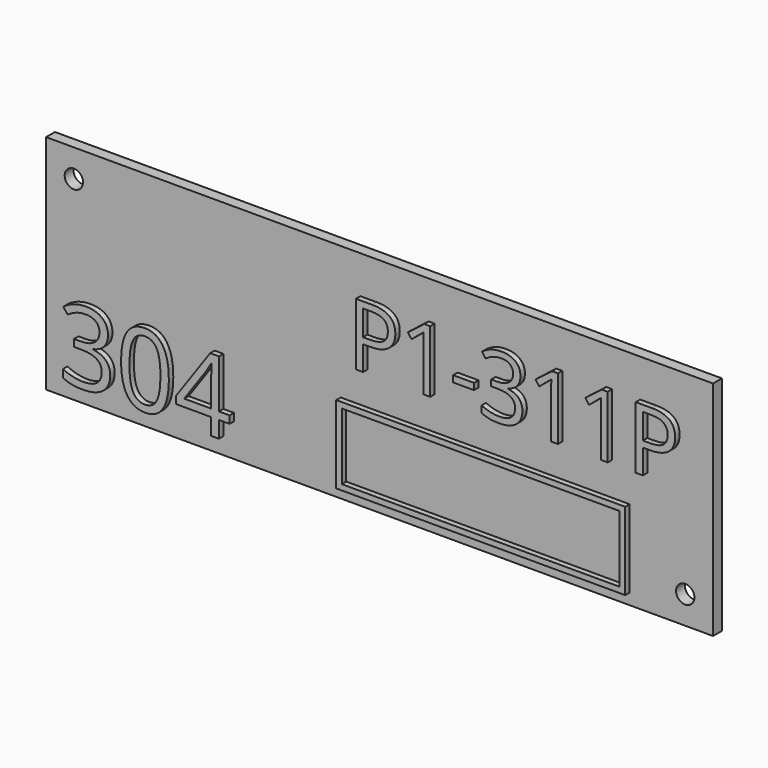
from build123d import *

# Parameters (mm, degrees)
F0_W         = 120
F0_H         = 40
F1_DEPTH     = 2
F3_D         = 3.3
F4_TEXT_SIZE = 15.681149951
F5_DEPTH     = 1
F6_TEXT_SIZE = 18.1818181818
F7_DEPTH     = 1
F8_W         = 52
F8_H         = 14
F8_W_2       = 49.99999962
F8_H_2       = 11.99999962
F9_DEPTH     = 1


# Not quite as in the source:
# - Text() gives the source's letters only with a copy of the font that has no kerning and outlines rounded to 1/6400 em; it was checked with that copy


with BuildPart() as f1:
    # F0 (on Front) → F1 (new body)
    with BuildSketch(Plane.XZ):
        Rectangle(F0_W, F0_H)
    extrude(amount=F1_DEPTH)

    # F3 (through all)
    with Locations(Plane.XZ.offset(2)):
        with Locations((-55, 15), (55, -15)):
            Hole(F3_D / 2)

    # F4 (on face) → F5 (join)
    with BuildSketch(Plane.XZ.offset(2)):
        with Locations((-5, 2)):
            Text('P1-311P', F4_TEXT_SIZE, font='Open Sans', text_align=(TextAlign.LEFT, TextAlign.BOTTOM))
    extrude(amount=F5_DEPTH)

    # F6 (on face) → F7 (join)
    with BuildSketch(Plane.XZ.offset(2)):
        with Locations((-57, -17)):
            Text('304', F6_TEXT_SIZE, font='Open Sans', text_align=(TextAlign.LEFT, TextAlign.BOTTOM))
    extrude(amount=F7_DEPTH)

    # F8 (on face) → F9 (join)
    with BuildSketch(Plane.XZ.offset(2)):
        with Locations((19, -11)):
            Rectangle(F8_W, F8_H)
        with Locations((19, -11)):
            Rectangle(F8_W_2, F8_H_2, mode=Mode.SUBTRACT)
    extrude(amount=F9_DEPTH)


solid = f1.part
